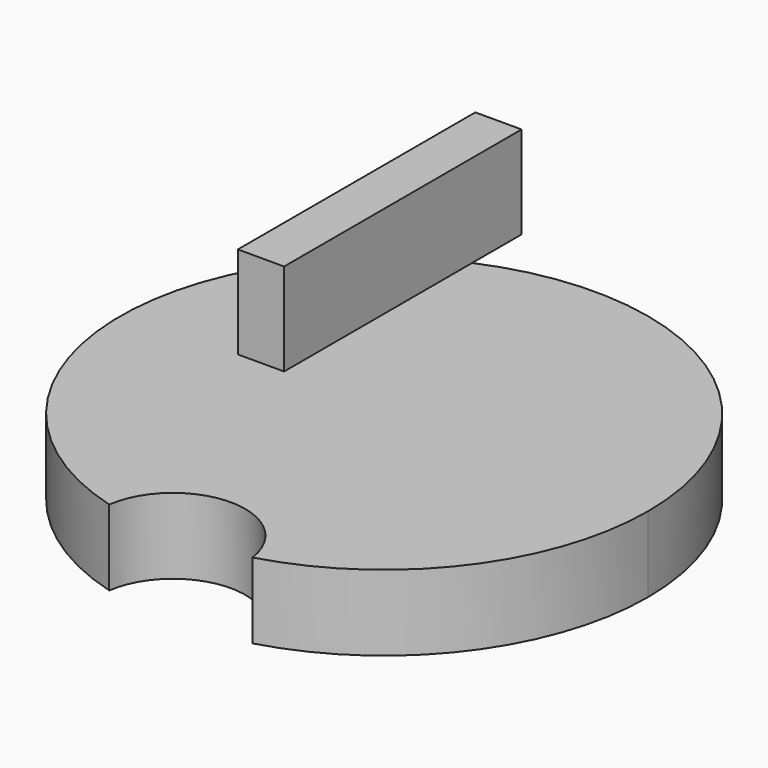
from build123d import *

# Parameters (mm, degrees)
F3_DEPTH = 27.432
F5_DEPTH = 33.528


# Not quite as in the source:
# - the program builds the solid bodies; features that only make, move or delete a surface that nothing else refers to are left out


with BuildPart() as f3:
    # F2 (on Top) → F3 (new body)
    with BuildSketch(Plane.XY):
        with BuildLine():
            ThreePointArc((25.9753267238, -94.6690976426), (76.334874565, -60.3082301144), (95.7446020854, -2.515360713))
            ThreePointArc((95.7446020854, -2.515360713), (-57.7928694014, 73.819513852), (-25.9753267238, -94.6690976426))
            ThreePointArc((-25.9753267238, -94.6690976426), (0, -72.0376076224), (25.9753267238, -94.6690976426))
        make_face()
    extrude(amount=F3_DEPTH)

    # F4 (on face) → F5 (join)
    with BuildSketch(Plane.XY.offset(27.432)):
        with BuildLine():
            ThreePointArc((-55.0617836416, 75.8123407131), (-46.9138023818, 80.9479484388), (-38.2910855114, 85.23896453))
            Line((-38.2910855114, 85.23896453), (-38.2910855114, 107.650950551))
            Line((-38.2910855114, 107.650950551), (-55.0617836416, 107.650950551))
            Line((-55.0617836416, 107.650950551), (-55.0617836416, 75.8123407131))
        make_face()
        with BuildLine():
            Line((-55.0617836416, 0), (-38.2910855114, 0))
            Line((-38.2910855114, 0), (-38.2910855114, 85.23896453))
            ThreePointArc((-38.2910855114, 85.23896453), (-46.9138023818, 80.9479484388), (-55.0617836416, 75.8123407131))
            Line((-55.0617836416, 75.8123407131), (-55.0617836416, 0))
        make_face()
    extrude(amount=F5_DEPTH)


solid = f3.part
